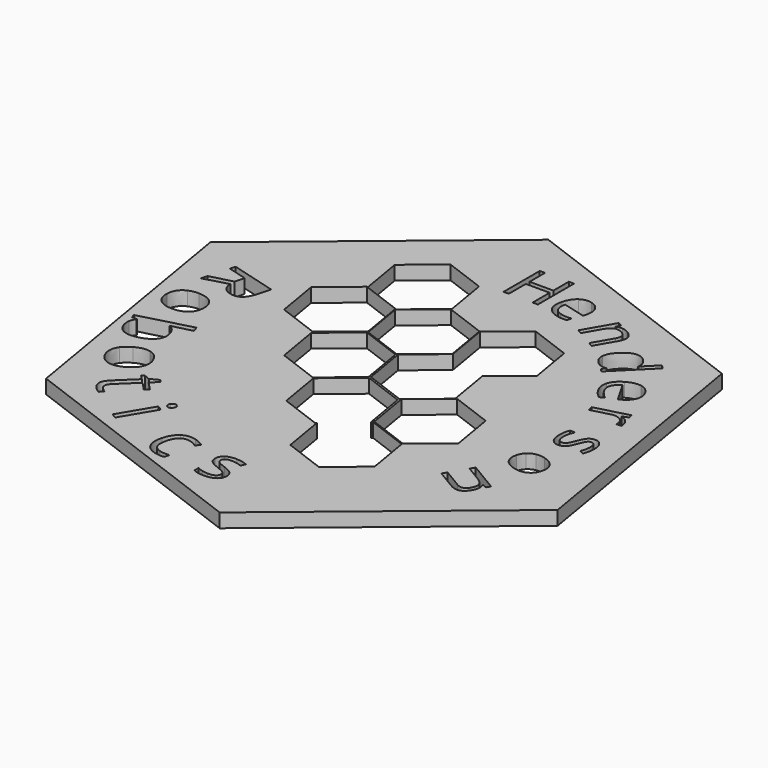
from build123d import *

# Parameters (mm, degrees)
F1_DEPTH = 6.35


with BuildPart() as f1:
    # F0 (on Top) → F1 (new body)
    with BuildSketch(Plane.XY):
        Polygon((112.5371310165, -18.0102200831), (92.5793495724, 100.4138352002), (-19.9577814441, 142.341917108), (-112.5371310165, 65.8459437326), (-92.5793495724, -52.5781115507), (19.9577814441, -94.5061934585), align=None)
        with BuildLine():
            add(Edge.make_bspline(
                [(-72.967737569, -43.6153682612), (-73.0631727177, -44.8083966458), (-72.1048965995, -45.8071760261)],
                knots=[0, 0, 0, 1, 1, 1], degree=2))
            add(Edge.make_bspline(
                [(-72.1048965995, -45.8071760261), (-71.5883258796, -46.3455805358), (-71.0311581814, -46.7701049042)],
                knots=[0, 0, 0, 1, 1, 1], degree=2))
            add(Edge.make_bspline(
                [(-71.0311581814, -46.7701049042), (-70.4739904832, -47.1946292726), (-70.1074129237, -47.4048885653)],
                knots=[0, 0, 0, 1, 1, 1], degree=2))
            Line((-70.1074129237, -47.4048885653), (-71.6563012596, -48.8909652017))
            add(Edge.make_bspline(
                [(-71.6563012596, -48.8909652017), (-72.126794889, -48.712971361), (-72.84603054, -48.1741965048)],
                knots=[0, 0, 0, 1, 1, 1], degree=2))
            add(Edge.make_bspline(
                [(-72.84603054, -48.1741965048), (-73.565266191, -47.6354216486), (-74.0593773144, -47.1204260307)],
                knots=[0, 0, 0, 1, 1, 1], degree=2))
            add(Edge.make_bspline(
                [(-74.0593773144, -47.1204260307), (-77.7764405384, -43.24625445), (-73.6915889323, -39.3270548574)],
                knots=[0, 0, 0, 1, 1, 1], degree=2))
            Line((-73.6915889323, -39.3270548574), (-65.7403687094, -31.6982785728))
            Line((-65.7403687094, -31.6982785728), (-67.5783123579, -29.7826509333))
            Line((-67.5783123579, -29.7826509333), (-66.6029418693, -28.8468344116))
            Line((-66.6029418693, -28.8468344116), (-63.9222781187, -29.9539165765))
            Line((-63.9222781187, -29.9539165765), (-60.2542628032, -28.0681121332))
            Line((-60.2542628032, -28.0681121332), (-59.1312829772, -29.2385567195))
            Line((-59.1312829772, -29.2385567195), (-62.2290596489, -32.2107099923))
            Line((-62.2290596489, -32.2107099923), (-58.5082531589, -36.0887830548))
            Line((-58.5082531589, -36.0887830548), (-60.0805503864, -37.5973192877))
            Line((-60.0805503864, -37.5973192877), (-63.8013568765, -33.7192462252))
            Line((-63.8013568765, -33.7192462252), (-71.6667444964, -41.2656706558))
            add(Edge.make_bspline(
                [(-71.6667444964, -41.2656706558), (-72.8723024203, -42.4223398765), (-72.967737569, -43.6153682612)],
                knots=[0, 0, 0, 1, 1, 1], degree=2))
        make_face(mode=Mode.SUBTRACT)
        with BuildLine():
            add(Edge.make_bspline(
                [(3.4055142751, -68.3015490873), (4.4394744841, -69.3937738183), (4.435601775, -71.0454177006)],
                knots=[0, 0, 0, 1, 1, 1], degree=2))
            add(Edge.make_bspline(
                [(4.435601775, -71.0454177006), (4.4301731682, -73.3606252541), (2.7029292089, -74.6134783422)],
                knots=[0, 0, 0, 1, 1, 1], degree=2))
            add(Edge.make_bspline(
                [(2.7029292089, -74.6134783422), (0.9756852496, -75.8663314303), (-2.143548358, -75.859017575)],
                knots=[0, 0, 0, 1, 1, 1], degree=2))
            add(Edge.make_bspline(
                [(-2.143548358, -75.859017575), (-5.4419925922, -75.8512835138), (-7.2849245981, -74.8007539515)],
                knots=[0, 0, 0, 1, 1, 1], degree=2))
            Line((-7.2849245981, -74.8007539515), (-7.2794619205, -72.4710158066))
            add(Edge.make_bspline(
                [(-7.2794619205, -72.4710158066), (-6.0845295149, -73.0792622713), (-4.7170441834, -73.4287830276)],
                knots=[0, 0, 0, 1, 1, 1], degree=2))
            add(Edge.make_bspline(
                [(-4.7170441834, -73.4287830276), (-3.3495588518, -73.7783037839), (-2.0757103443, -73.7812906533)],
                knots=[0, 0, 0, 1, 1, 1], degree=2))
            add(Edge.make_bspline(
                [(-2.0757103443, -73.7812906533), (-0.109236983, -73.7859015621), (0.9505451405, -73.1611458558)],
                knots=[0, 0, 0, 1, 1, 1], degree=2))
            add(Edge.make_bspline(
                [(0.9505451405, -73.1611458558), (2.010327264, -72.5363901496), (2.0133482042, -71.2480110508)],
                knots=[0, 0, 0, 1, 1, 1], degree=2))
            add(Edge.make_bspline(
                [(2.0133482042, -71.2480110508), (2.0156195878, -70.2793049614), (1.1793015029, -69.5895588912)],
                knots=[0, 0, 0, 1, 1, 1], degree=2))
            add(Edge.make_bspline(
                [(1.1793015029, -69.5895588912), (0.342983418, -68.8998128209), (-2.095952685, -67.9544440275)],
                knots=[0, 0, 0, 1, 1, 1], degree=2))
            add(Edge.make_bspline(
                [(-2.095952685, -67.9544440275), (-4.4091387071, -67.0868670012), (-5.383599622, -66.4403890328)],
                knots=[0, 0, 0, 1, 1, 1], degree=2))
            add(Edge.make_bspline(
                [(-5.383599622, -66.4403890328), (-6.3580605369, -65.7939110644), (-6.8332346452, -64.9766575277)],
                knots=[0, 0, 0, 1, 1, 1], degree=2))
            add(Edge.make_bspline(
                [(-6.8332346452, -64.9766575277), (-7.3084087535, -64.159403991), (-7.3057512346, -63.0260178664)],
                knots=[0, 0, 0, 1, 1, 1], degree=2))
            add(Edge.make_bspline(
                [(-7.3057512346, -63.0260178664), (-7.3009926859, -60.9965786093), (-5.646594751, -59.825895185)],
                knots=[0, 0, 0, 1, 1, 1], degree=2))
            add(Edge.make_bspline(
                [(-5.646594751, -59.825895185), (-3.992196816, -58.6552117608), (-1.1199832611, -58.6619464132)],
                knots=[0, 0, 0, 1, 1, 1], degree=2))
            add(Edge.make_bspline(
                [(-1.1199832611, -58.6619464132), (1.5584890759, -58.6682267889), (4.1181613756, -59.7640289491)],
                knots=[0, 0, 0, 1, 1, 1], degree=2))
            Line((4.1181613756, -59.7640289491), (3.2173156235, -61.8058977678))
            add(Edge.make_bspline(
                [(3.2173156235, -61.8058977678), (0.7253051101, -60.7732205003), (-1.3041341471, -60.7684619516)],
                knots=[0, 0, 0, 1, 1, 1], degree=2))
            add(Edge.make_bspline(
                [(-1.3041341471, -60.7684619516), (-3.0913968819, -60.7642712488), (-4.0008705647, -61.3215695932)],
                knots=[0, 0, 0, 1, 1, 1], degree=2))
            add(Edge.make_bspline(
                [(-4.0008705647, -61.3215695932), (-4.9103442475, -61.8788679377), (-4.9126497018, -62.8621046184)],
                knots=[0, 0, 0, 1, 1, 1], degree=2))
            add(Edge.make_bspline(
                [(-4.9126497018, -62.8621046184), (-4.9142169565, -63.53051182), (-4.5738440026, -63.9987131708)],
                knots=[0, 0, 0, 1, 1, 1], degree=2))
            add(Edge.make_bspline(
                [(-4.5738440026, -63.9987131708), (-4.2334710488, -64.4669145217), (-3.4788740294, -64.892495115)],
                knots=[0, 0, 0, 1, 1, 1], degree=2))
            add(Edge.make_bspline(
                [(-3.4788740294, -64.892495115), (-2.7242770101, -65.3180757083), (-0.5756347401, -66.1271442341)],
                knots=[0, 0, 0, 1, 1, 1], degree=2))
            add(Edge.make_bspline(
                [(-0.5756347401, -66.1271442341), (2.3715540661, -67.2093243564), (3.4055142751, -68.3015490873)],
                knots=[0, 0, 0, 1, 1, 1], degree=2))
        make_face(mode=Mode.SUBTRACT)
        Polygon((-45.7921878886, -45.7525988365), (-54.6549116375, -60.6645132283), (-56.9145564752, -59.3215194689), (-48.0518327263, -44.4096050772), align=None, mode=Mode.SUBTRACT)
        with BuildLine():
            add(Edge.make_bspline(
                [(-46.1364735974, -41.6181544447), (-46.294896449, -41.0173039437), (-45.8420565495, -40.2553813106)],
                knots=[0, 0, 0, 1, 1, 1], degree=2))
            add(Edge.make_bspline(
                [(-45.8420565495, -40.2553813106), (-45.3814536802, -39.4803971466), (-44.7857168684, -39.3454480761)],
                knots=[0, 0, 0, 1, 1, 1], degree=2))
            add(Edge.make_bspline(
                [(-44.7857168684, -39.3454480761), (-44.1899800566, -39.2104990056), (-43.615272699, -39.5520696727)],
                knots=[0, 0, 0, 1, 1, 1], degree=2))
            add(Edge.make_bspline(
                [(-43.615272699, -39.5520696727), (-43.0710422467, -39.8755267438), (-42.8956763794, -40.477609449)],
                knots=[0, 0, 0, 1, 1, 1], degree=2))
            add(Edge.make_bspline(
                [(-42.8956763794, -40.477609449), (-42.720310512, -41.0796921542), (-43.1731504116, -41.8416147874)],
                knots=[0, 0, 0, 1, 1, 1], degree=2))
            add(Edge.make_bspline(
                [(-43.1731504116, -41.8416147874), (-43.6259903112, -42.6035374206), (-44.2425516236, -42.7437850522)],
                knots=[0, 0, 0, 1, 1, 1], degree=2))
            add(Edge.make_bspline(
                [(-44.2425516236, -42.7437850522), (-44.8591129359, -42.8840326839), (-45.4033433882, -42.5605756127)],
                knots=[0, 0, 0, 1, 1, 1], degree=2))
            add(Edge.make_bspline(
                [(-45.4033433882, -42.5605756127), (-45.9780507458, -42.2190049456), (-46.1364735974, -41.6181544447)],
                knots=[0, 0, 0, 1, 1, 1], degree=2))
        make_face(mode=Mode.SUBTRACT)
        with BuildLine():
            add(Edge.make_bspline(
                [(-22.1531029202, -73.3679597217), (-24.046773454, -73.7883237584), (-26.5742108863, -73.109078064)],
                knots=[0, 0, 0, 1, 1, 1], degree=2))
            add(Edge.make_bspline(
                [(-26.5742108863, -73.109078064), (-30.1765355025, -72.1409577638), (-31.5560373116, -69.3924930371)],
                knots=[0, 0, 0, 1, 1, 1], degree=2))
            add(Edge.make_bspline(
                [(-31.5560373116, -69.3924930371), (-32.9355391206, -66.6440283103), (-31.845102546, -62.5865712829)],
                knots=[0, 0, 0, 1, 1, 1], degree=2))
            add(Edge.make_bspline(
                [(-31.845102546, -62.5865712829), (-30.7273399952, -58.4274357382), (-28.1101195997, -56.6959782374)],
                knots=[0, 0, 0, 1, 1, 1], degree=2))
            add(Edge.make_bspline(
                [(-28.1101195997, -56.6959782374), (-25.4928992043, -54.9645207366), (-21.7888960707, -55.9599670129)],
                knots=[0, 0, 0, 1, 1, 1], degree=2))
            add(Edge.make_bspline(
                [(-21.7888960707, -55.9599670129), (-20.5929630328, -56.2813725427), (-19.4666461724, -56.8618162001)],
                knots=[0, 0, 0, 1, 1, 1], degree=2))
            add(Edge.make_bspline(
                [(-19.4666461724, -56.8618162001), (-18.340329312, -57.4422598575), (-17.7561615907, -57.9730450919)],
                knots=[0, 0, 0, 1, 1, 1], degree=2))
            Line((-17.7561615907, -57.9730450919), (-19.0985574859, -59.8965554459))
            add(Edge.make_bspline(
                [(-19.0985574859, -59.8965554459), (-19.8415676113, -59.3386561312), (-20.7659042827, -58.8566224905)],
                knots=[0, 0, 0, 1, 1, 1], degree=2))
            add(Edge.make_bspline(
                [(-20.7659042827, -58.8566224905), (-21.6902409542, -58.3745888499), (-22.4455670834, -58.1715958837)],
                knots=[0, 0, 0, 1, 1, 1], degree=2))
            add(Edge.make_bspline(
                [(-22.4455670834, -58.1715958837), (-27.5004419481, -56.8131044948), (-29.2323883453, -63.2575857638)],
                knots=[0, 0, 0, 1, 1, 1], degree=2))
            add(Edge.make_bspline(
                [(-29.2323883453, -63.2575857638), (-30.0534688687, -66.3127831198), (-29.2603895494, -68.2780669563)],
                knots=[0, 0, 0, 1, 1, 1], degree=2))
            add(Edge.make_bspline(
                [(-29.2603895494, -68.2780669563), (-28.4673102302, -70.2433507928), (-26.0463931494, -70.8939692741)],
                knots=[0, 0, 0, 1, 1, 1], degree=2))
            add(Edge.make_bspline(
                [(-26.0463931494, -70.8939692741), (-23.9740881282, -71.4508986941), (-21.5558351544, -71.1455578415)],
                knots=[0, 0, 0, 1, 1, 1], degree=2))
            Line((-21.5558351544, -71.1455578415), (-22.1531029202, -73.3679597217))
        make_face(mode=Mode.SUBTRACT)
        with BuildLine():
            add(Edge.make_bspline(
                [(-71.4948339907, -23.0783226482), (-72.561892733, -26.0609442778), (-76.1022720551, -28.0076234528)],
                knots=[0, 0, 0, 1, 1, 1], degree=2))
            add(Edge.make_bspline(
                [(-76.1022720551, -28.0076234528), (-79.7425639224, -30.0092395861), (-82.7932065522, -29.3020526751)],
                knots=[0, 0, 0, 1, 1, 1], degree=2))
            add(Edge.make_bspline(
                [(-82.7932065522, -29.3020526751), (-85.843849182, -28.5948657642), (-87.6209403553, -25.3629121254)],
                knots=[0, 0, 0, 1, 1, 1], degree=2))
            add(Edge.make_bspline(
                [(-87.6209403553, -25.3629121254), (-88.7196795215, -23.3646612196), (-88.6316989727, -21.3022590841)],
                knots=[0, 0, 0, 1, 1, 1], degree=2))
            add(Edge.make_bspline(
                [(-88.6316989727, -21.3022590841), (-88.5437184239, -19.2398569486), (-87.2564581701, -17.4345252971)],
                knots=[0, 0, 0, 1, 1, 1], degree=2))
            add(Edge.make_bspline(
                [(-87.2564581701, -17.4345252971), (-85.9691979163, -15.6291936455), (-83.6190810902, -14.3369808435)],
                knots=[0, 0, 0, 1, 1, 1], degree=2))
            add(Edge.make_bspline(
                [(-83.6190810902, -14.3369808435), (-79.9831332465, -12.3377532736), (-76.9514940964, -13.0412458155)],
                knots=[0, 0, 0, 1, 1, 1], degree=2))
            add(Edge.make_bspline(
                [(-76.9514940964, -13.0412458155), (-73.9198549462, -13.7447383575), (-72.142763773, -16.9766919963)],
                knots=[0, 0, 0, 1, 1, 1], degree=2))
            add(Edge.make_bspline(
                [(-72.142763773, -16.9766919963), (-70.4277752483, -20.0957010186), (-71.4948339907, -23.0783226482)],
                knots=[0, 0, 0, 1, 1, 1], degree=2))
        make_face(mode=Mode.SUBTRACT)
        with BuildLine():
            Line((-74.547481639, 8.9194912074), (-75.7870057133, 8.5857765521))
            Line((-75.7870057133, 8.5857765521), (-80.2644527998, 7.3803221831))
            add(Edge.make_bspline(
                [(-80.2644527998, 7.3803221831), (-82.1846199325, 6.8633593213), (-83.7407325732, 6.5740920086)],
                knots=[0, 0, 0, 1, 1, 1], degree=2))
            Line((-83.7407325732, 6.5740920086), (-83.7081782368, 6.4531746829))
            add(Edge.make_bspline(
                [(-83.7081782368, 6.4531746829), (-80.7604046149, 5.3690046154), (-79.8319549412, 1.9204424854)],
                knots=[0, 0, 0, 1, 1, 1], degree=2))
            add(Edge.make_bspline(
                [(-79.8319549412, 1.9204424854), (-78.9529878588, -1.3443253095), (-80.6963415598, -3.751132119)],
                knots=[0, 0, 0, 1, 1, 1], degree=2))
            add(Edge.make_bspline(
                [(-80.6963415598, -3.751132119), (-82.4396952609, -6.1579389284), (-86.5170274847, -7.2556711513)],
                knots=[0, 0, 0, 1, 1, 1], degree=2))
            add(Edge.make_bspline(
                [(-86.5170274847, -7.2556711513), (-90.5991964016, -8.3547055476), (-93.3506186988, -7.1424567124)],
                knots=[0, 0, 0, 1, 1, 1], degree=2))
            add(Edge.make_bspline(
                [(-93.3506186988, -7.1424567124), (-96.102040996, -5.9302078772), (-96.9731950376, -2.6944602404)],
                knots=[0, 0, 0, 1, 1, 1], degree=2))
            add(Edge.make_bspline(
                [(-96.9731950376, -2.6944602404), (-97.4094231452, -1.0741680756), (-97.1721425165, 0.4239959688)],
                knots=[0, 0, 0, 1, 1, 1], degree=2))
            add(Edge.make_bspline(
                [(-97.1721425165, 0.4239959688), (-96.9348618877, 1.9221600132), (-95.9353382153, 3.1612801877)],
                knots=[0, 0, 0, 1, 1, 1], degree=2))
            Line((-95.9353382153, 3.1612801877), (-95.9848208066, 3.3450745229))
            Line((-95.9848208066, 3.3450745229), (-98.2597393392, 3.2980155693))
            Line((-98.2597393392, 3.2980155693), (-98.7441478646, 5.0972653762))
            Line((-98.7441478646, 5.0972653762), (-76.4598394845, 11.0968263711))
            Line((-76.4598394845, 11.0968263711), (-75.2233096623, 11.4297348897))
            Line((-75.2233096623, 11.4297348897), (-74.547481639, 8.9194912074))
        make_face(mode=Mode.SUBTRACT)
        Polygon((-3.2903466672, 19.5115212872), (15.2522997676, 12.6052844447), (18.4983979383, -6.6438464109), (19.0837242934, -6.1601026273), (37.6263707282, -13.0663394699), (40.9167173954, -32.5778607571), (25.6644176278, -45.1831452018), (7.121771193, -38.2769083592), (3.8756730223, -19.0277775036), (3.2903466672, -19.5115212872), (-15.2522997676, -12.6052844447), (-18.5426464348, 6.9062368426), align=None, mode=Mode.SUBTRACT)
        Polygon((49.7063692499, 19.6015298515), (52.9967159171, 0.0900085643), (37.7444161495, -12.5152758804), (19.2017697146, -5.6090390378), (15.9114230474, 13.9024822494), (31.1637228151, 26.5077666941), align=None, mode=Mode.SUBTRACT)
        with BuildLine():
            Line((62.722350632, -21.8460348177), (63.9337989853, -19.8183676586))
            Line((63.9337989853, -19.8183676586), (72.5914298611, -24.9909486816))
            add(Edge.make_bspline(
                [(72.5914298611, -24.9909486816), (74.2245028331, -25.9666431165), (75.4759367053, -25.7043955079)],
                knots=[0, 0, 0, 1, 1, 1], degree=2))
            add(Edge.make_bspline(
                [(75.4759367053, -25.7043955079), (76.7273705775, -25.4421478993), (77.677388843, -23.8520505318)],
                knots=[0, 0, 0, 1, 1, 1], degree=2))
            add(Edge.make_bspline(
                [(77.677388843, -23.8520505318), (78.9308527461, -21.7540596562), (78.3794554024, -20.0992570813)],
                knots=[0, 0, 0, 1, 1, 1], degree=2))
            add(Edge.make_bspline(
                [(78.3794554024, -20.0992570813), (77.8280580587, -18.4444545063), (75.2143599288, -16.8828765711)],
                knots=[0, 0, 0, 1, 1, 1], degree=2))
            Line((75.2143599288, -16.8828765711), (68.1937088982, -12.6883241802))
            Line((68.1937088982, -12.6883241802), (69.4051572515, -10.6606570211))
            Line((69.4051572515, -10.6606570211), (82.7861977522, -18.655282474))
            Line((82.7861977522, -18.655282474), (81.8011665285, -20.3039829387))
            Line((81.8011665285, -20.3039829387), (79.7727704605, -19.5374217896))
            Line((79.7727704605, -19.5374217896), (79.7144155302, -19.6350936181))
            add(Edge.make_bspline(
                [(79.7144155302, -19.6350936181), (80.3293828803, -20.8507452151), (80.2033099846, -22.2995917537)],
                knots=[0, 0, 0, 1, 1, 1], degree=2))
            add(Edge.make_bspline(
                [(80.2033099846, -22.2995917537), (80.0772370888, -23.7484382923), (79.2532654728, -25.1275645103)],
                knots=[0, 0, 0, 1, 1, 1], degree=2))
            add(Edge.make_bspline(
                [(79.2532654728, -25.1275645103), (77.8083973983, -27.5459189833), (75.9127591374, -28.0700589712)],
                knots=[0, 0, 0, 1, 1, 1], degree=2))
            add(Edge.make_bspline(
                [(75.9127591374, -28.0700589712), (74.0171208765, -28.5941989592), (71.4503052243, -27.0606313905)],
                knots=[0, 0, 0, 1, 1, 1], degree=2))
            Line((71.4503052243, -27.0606313905), (62.722350632, -21.8460348177))
        make_face(mode=Mode.SUBTRACT)
        with BuildLine():
            add(Edge.make_bspline(
                [(86.1770568848, -2.2785955218), (83.7359495083, -3.4962546919), (80.3751698675, -2.5957365013)],
                knots=[0, 0, 0, 1, 1, 1], degree=2))
            add(Edge.make_bspline(
                [(80.3751698675, -2.5957365013), (76.9195461387, -1.6698049138), (75.4450941098, 0.5881857946)],
                knots=[0, 0, 0, 1, 1, 1], degree=2))
            add(Edge.make_bspline(
                [(75.4450941098, 0.5881857946), (73.9706420808, 2.8461765029), (74.7927102205, 5.9141765676)],
                knots=[0, 0, 0, 1, 1, 1], degree=2))
            add(Edge.make_bspline(
                [(74.7927102205, 5.9141765676), (75.3009781564, 7.811058328), (76.5850430377, 9.0404149205)],
                knots=[0, 0, 0, 1, 1, 1], degree=2))
            add(Edge.make_bspline(
                [(76.5850430377, 9.0404149205), (77.869107919, 10.2697715131), (79.7452977647, 10.6244738683)],
                knots=[0, 0, 0, 1, 1, 1], degree=2))
            add(Edge.make_bspline(
                [(79.7452977647, 10.6244738683), (81.6214876104, 10.9791762234), (83.8523855069, 10.3814089337)],
                knots=[0, 0, 0, 1, 1, 1], degree=2))
            add(Edge.make_bspline(
                [(83.8523855069, 10.3814089337), (87.3038855796, 9.4565822765), (88.7687289663, 7.212215499)],
                knots=[0, 0, 0, 1, 1, 1], degree=2))
            add(Edge.make_bspline(
                [(88.7687289663, 7.212215499), (90.233572353, 4.9678487216), (89.4115042133, 1.8998486569)],
                knots=[0, 0, 0, 1, 1, 1], degree=2))
            add(Edge.make_bspline(
                [(89.4115042133, 1.8998486569), (88.6181642613, -1.0609363518), (86.1770568848, -2.2785955218)],
                knots=[0, 0, 0, 1, 1, 1], degree=2))
        make_face(mode=Mode.SUBTRACT)
        with BuildLine():
            add(Edge.make_bspline(
                [(-85.1180984879, 19.3300737728), (-87.4584878856, 17.3235839335), (-91.3898794736, 17.3855591027)],
                knots=[0, 0, 0, 1, 1, 1], degree=2))
            add(Edge.make_bspline(
                [(-91.3898794736, 17.3855591027), (-95.432218309, 17.4492832644), (-97.669760896, 19.5182904687)],
                knots=[0, 0, 0, 1, 1, 1], degree=2))
            add(Edge.make_bspline(
                [(-97.669760896, 19.5182904687), (-99.9073034829, 21.587297673), (-99.8507273775, 25.1761999325)],
                knots=[0, 0, 0, 1, 1, 1], degree=2))
            add(Edge.make_bspline(
                [(-99.8507273775, 25.1761999325), (-99.8157475274, 27.395144878), (-98.7467367995, 29.0959899931)],
                knots=[0, 0, 0, 1, 1, 1], degree=2))
            add(Edge.make_bspline(
                [(-98.7467367995, 29.0959899931), (-97.6777260716, 30.7968351082), (-95.7189849761, 31.7020056295)],
                knots=[0, 0, 0, 1, 1, 1], degree=2))
            add(Edge.make_bspline(
                [(-95.7189849761, 31.7020056295), (-93.7602438806, 32.6071761509), (-91.150571673, 32.5660368054)],
                knots=[0, 0, 0, 1, 1, 1], degree=2))
            add(Edge.make_bspline(
                [(-91.150571673, 32.5660368054), (-87.113056631, 32.5023886868), (-84.8897953163, 30.4456690954)],
                knots=[0, 0, 0, 1, 1, 1], degree=2))
            add(Edge.make_bspline(
                [(-84.8897953163, 30.4456690954), (-82.6665340015, 28.388949504), (-82.7231101069, 24.8000472444)],
                knots=[0, 0, 0, 1, 1, 1], degree=2))
            add(Edge.make_bspline(
                [(-82.7231101069, 24.8000472444), (-82.7777090903, 21.3365636122), (-85.1180984879, 19.3300737728)],
                knots=[0, 0, 0, 1, 1, 1], degree=2))
        make_face(mode=Mode.SUBTRACT)
        with BuildLine():
            Line((-86.9551316498, 47.5102251238), (-85.7417407996, 51.8623928649))
            Line((-85.7417407996, 51.8623928649), (-94.4095801162, 54.2789993801))
            Line((-94.4095801162, 54.2789993801), (-93.7342021901, 56.701432368))
            Line((-93.7342021901, 56.701432368), (-72.890329644, 50.8901296482))
            Line((-72.890329644, 50.8901296482), (-74.4840180458, 45.1739177199))
            add(Edge.make_bspline(
                [(-74.4840180458, 45.1739177199), (-75.5536844033, 41.3372583172), (-77.53332218, 39.9151582183)],
                knots=[0, 0, 0, 1, 1, 1], degree=2))
            add(Edge.make_bspline(
                [(-77.53332218, 39.9151582183), (-79.5129599567, 38.4930581195), (-82.4645873451, 39.3159762328)],
                knots=[0, 0, 0, 1, 1, 1], degree=2))
            add(Edge.make_bspline(
                [(-82.4645873451, 39.3159762328), (-86.5977780929, 40.4683159711), (-86.8841882796, 45.0665485028)],
                knots=[0, 0, 0, 1, 1, 1], degree=2))
            Line((-86.8841882796, 45.0665485028), (-97.828442386, 42.0162877574))
            Line((-97.828442386, 42.0162877574), (-97.0296903379, 44.8812367525))
            Line((-97.0296903379, 44.8812367525), (-86.9551316498, 47.5102251238))
        make_face(mode=Mode.SUBTRACT)
        Polygon((-3.8754936377, 19.9034995977), (-19.1277934053, 7.2982151531), (-37.6704398402, 14.2044519956), (-40.9607865074, 33.7159732829), (-25.7084867398, 46.3212577275), (-7.1658403049, 39.415020885), align=None, mode=Mode.SUBTRACT)
        Polygon((-29.1757911749, 66.8978677121), (-25.8854445077, 47.3863464248), (-41.1377442753, 34.7810619802), (-59.6803907101, 41.6872988227), (-62.9707373774, 61.19882011), (-47.7184376097, 73.8041045547), align=None, mode=Mode.SUBTRACT)
        Polygon((4.9981049395, 71.9796337144), (8.2884516067, 52.4681124272), (-6.9638481609, 39.8628279825), (-25.5064945957, 46.7690648251), (-28.7968412629, 66.2805861123), (-13.5445414953, 78.885870557), align=None, mode=Mode.SUBTRACT)
        Polygon((-16.7064143599, 98.8550308269), (-13.4160676927, 79.3435095397), (-28.6683674603, 66.738225095), (-47.2110138952, 73.6444619376), (-50.5013605624, 93.1559832248), (-35.2490607947, 105.7612676695), align=None, mode=Mode.SUBTRACT)
        Polygon((27.3264721896, 45.6410835091), (30.6145172825, 26.1432103934), (15.3622175149, 13.5379259488), (-3.1804289199, 20.4441627913), (-6.4707755871, 39.9556840786), (8.558592322, 52.3767261775), (5.2705472291, 71.8745992932), (20.5228469967, 84.4798837378), (39.0654934316, 77.5736468953), (42.3558400988, 58.062125608), align=None, mode=Mode.SUBTRACT)
        with BuildLine():
            add(Edge.make_bspline(
                [(88.0708640482, 50.9387753988), (89.1739242686, 49.9801827882), (89.5492388219, 48.5794898066)],
                knots=[0, 0, 0, 1, 1, 1], degree=2))
            add(Edge.make_bspline(
                [(89.5492388219, 48.5794898066), (89.8149894993, 47.5876947762), (89.8606590671, 46.7560569418)],
                knots=[0, 0, 0, 1, 1, 1], degree=2))
            Line((89.8606590671, 46.7560569418), (87.6843982847, 46.5086146889))
            add(Edge.make_bspline(
                [(87.6843982847, 46.5086146889), (87.6417457531, 47.4855920059), (87.4517573302, 48.1946384531)],
                knots=[0, 0, 0, 1, 1, 1], degree=2))
            add(Edge.make_bspline(
                [(87.4517573302, 48.1946384531), (86.9668789012, 50.0042293858), (85.1549171792, 50.8940920188)],
                knots=[0, 0, 0, 1, 1, 1], degree=2))
            add(Edge.make_bspline(
                [(85.1549171792, 50.8940920188), (83.3429554572, 51.7839546518), (81.1549164208, 51.197671359)],
                knots=[0, 0, 0, 1, 1, 1], degree=2))
            Line((81.1549164208, 51.197671359), (73.1596564827, 49.0553479153))
            Line((73.1596564827, 49.0553479153), (72.5547240195, 51.312986603))
            Line((72.5547240195, 51.312986603), (87.4533993667, 55.3050746306))
            Line((87.4533993667, 55.3050746306), (87.9522646735, 53.4432839594))
            Line((87.9522646735, 53.4432839594), (85.2643128812, 52.4433118922))
            Line((85.2643128812, 52.4433118922), (85.2934522099, 52.3345624371))
            add(Edge.make_bspline(
                [(85.2934522099, 52.3345624371), (86.9678038278, 51.8973680094), (88.0708640482, 50.9387753988)],
                knots=[0, 0, 0, 1, 1, 1], degree=2))
        make_face(mode=Mode.SUBTRACT)
        with BuildLine():
            add(Edge.make_bspline(
                [(84.1783310039, 22.1919157172), (83.1275106211, 21.1924687754), (81.5349339521, 21.1924687754)],
                knots=[0, 0, 0, 1, 1, 1], degree=2))
            add(Edge.make_bspline(
                [(81.5349339521, 21.1924687754), (79.3025244277, 21.1924687754), (78.0905782529, 22.8551001366)],
                knots=[0, 0, 0, 1, 1, 1], degree=2))
            add(Edge.make_bspline(
                [(78.0905782529, 22.8551001366), (76.8786320781, 24.5177314978), (76.8786320781, 27.525412949)],
                knots=[0, 0, 0, 1, 1, 1], degree=2))
            add(Edge.make_bspline(
                [(76.8786320781, 27.525412949), (76.8786320781, 30.7058959742), (77.8874196456, 32.4852851557)],
                knots=[0, 0, 0, 1, 1, 1], degree=2))
            Line((77.8874196456, 32.4852851557), (80.1338401083, 32.4852851557))
            add(Edge.make_bspline(
                [(80.1338401083, 32.4852851557), (79.5500510068, 31.3317178911), (79.2161236407, 30.0123545216)],
                knots=[0, 0, 0, 1, 1, 1], degree=2))
            add(Edge.make_bspline(
                [(79.2161236407, 30.0123545216), (78.8821962746, 28.6929911521), (78.8821962746, 27.4646988824)],
                knots=[0, 0, 0, 1, 1, 1], degree=2))
            add(Edge.make_bspline(
                [(78.8821962746, 27.4646988824), (78.8821962746, 25.5685518806), (79.4870017838, 24.5480885311)],
                knots=[0, 0, 0, 1, 1, 1], degree=2))
            add(Edge.make_bspline(
                [(79.4870017838, 24.5480885311), (80.091807293, 23.5276251816), (81.3341105011, 23.5276251816)],
                knots=[0, 0, 0, 1, 1, 1], degree=2))
            add(Edge.make_bspline(
                [(81.3341105011, 23.5276251816), (82.2681730636, 23.5276251816), (82.931357483, 24.3355892981)],
                knots=[0, 0, 0, 1, 1, 1], degree=2))
            add(Edge.make_bspline(
                [(82.931357483, 24.3355892981), (83.5945419023, 25.1435534147), (84.5005825879, 27.4973910721)],
                knots=[0, 0, 0, 1, 1, 1], degree=2))
            add(Edge.make_bspline(
                [(84.5005825879, 27.4973910721), (85.3318982685, 29.7298005964), (85.9530498726, 30.6708686281)],
                knots=[0, 0, 0, 1, 1, 1], degree=2))
            add(Edge.make_bspline(
                [(85.9530498726, 30.6708686281), (86.5742014766, 31.6119366598), (87.3611491855, 32.0719624718)],
                knots=[0, 0, 0, 1, 1, 1], degree=2))
            add(Edge.make_bspline(
                [(87.3611491855, 32.0719624718), (88.1480968944, 32.5319882838), (89.2409500925, 32.5319882838)],
                knots=[0, 0, 0, 1, 1, 1], degree=2))
            add(Edge.make_bspline(
                [(89.2409500925, 32.5319882838), (91.1978111609, 32.5319882838), (92.3303620179, 30.9394116148)],
                knots=[0, 0, 0, 1, 1, 1], degree=2))
            add(Edge.make_bspline(
                [(92.3303620179, 30.9394116148), (93.4629128749, 29.3468349458), (93.4629128749, 26.5773394481)],
                knots=[0, 0, 0, 1, 1, 1], degree=2))
            add(Edge.make_bspline(
                [(93.4629128749, 26.5773394481), (93.4629128749, 23.9946564628), (92.4120924921, 21.5240609851)],
                knots=[0, 0, 0, 1, 1, 1], degree=2))
            Line((92.4120924921, 21.5240609851), (90.4412204853, 22.3880688554))
            add(Edge.make_bspline(
                [(90.4412204853, 22.3880688554), (91.4313268015, 24.7932799537), (91.4313268015, 26.7501410221)],
                knots=[0, 0, 0, 1, 1, 1], degree=2))
            add(Edge.make_bspline(
                [(91.4313268015, 26.7501410221), (91.4313268015, 28.4734864499), (90.8919056717, 29.3491701022)],
                knots=[0, 0, 0, 1, 1, 1], degree=2))
            add(Edge.make_bspline(
                [(90.8919056717, 29.3491701022), (90.3524845418, 30.2248537545), (89.4044110409, 30.2248537545)],
                knots=[0, 0, 0, 1, 1, 1], degree=2))
            add(Edge.make_bspline(
                [(89.4044110409, 30.2248537545), (88.7599078728, 30.2248537545), (88.3092226864, 29.8955967013)],
                knots=[0, 0, 0, 1, 1, 1], degree=2))
            add(Edge.make_bspline(
                [(88.3092226864, 29.8955967013), (87.8585375, 29.566339648), (87.4498851289, 28.8377708493)],
                knots=[0, 0, 0, 1, 1, 1], degree=2))
            add(Edge.make_bspline(
                [(87.4498851289, 28.8377708493), (87.0412327578, 28.1092020505), (86.265960831, 26.0355831618)],
                knots=[0, 0, 0, 1, 1, 1], degree=2))
            add(Edge.make_bspline(
                [(86.265960831, 26.0355831618), (85.2291513866, 23.1913626591), (84.1783310039, 22.1919157172)],
                knots=[0, 0, 0, 1, 1, 1], degree=2))
        make_face(mode=Mode.SUBTRACT)
        with BuildLine():
            add(Edge.make_bspline(
                [(67.8350967836, 60.6656310959), (67.0422062463, 61.5467535218), (66.2210770082, 62.9689910817)],
                knots=[0, 0, 0, 1, 1, 1], degree=2))
            add(Edge.make_bspline(
                [(66.2210770082, 62.9689910817), (64.4250046979, 66.0798795773), (65.2826695109, 68.9768716372)],
                knots=[0, 0, 0, 1, 1, 1], degree=2))
            add(Edge.make_bspline(
                [(65.2826695109, 68.9768716372), (66.1403343239, 71.8738636972), (69.5053401933, 73.8166507417)],
                knots=[0, 0, 0, 1, 1, 1], degree=2))
            add(Edge.make_bspline(
                [(69.5053401933, 73.8166507417), (72.9031354012, 75.7783687197), (75.8667133251, 75.2597162099)],
                knots=[0, 0, 0, 1, 1, 1], degree=2))
            add(Edge.make_bspline(
                [(75.8667133251, 75.2597162099), (78.830291249, 74.7410637002), (80.458351525, 71.9211805843)],
                knots=[0, 0, 0, 1, 1, 1], degree=2))
            add(Edge.make_bspline(
                [(80.458351525, 71.9211805843), (81.9799253004, 69.2857374978), (81.1315271957, 66.7465809638)],
                knots=[0, 0, 0, 1, 1, 1], degree=2))
            add(Edge.make_bspline(
                [(81.1315271957, 66.7465809638), (80.2831290909, 64.2074244298), (77.4386539711, 62.5651659537)],
                knots=[0, 0, 0, 1, 1, 1], degree=2))
            Line((77.4386539711, 62.5651659537), (76.0942910903, 61.7889976826))
            Line((76.0942910903, 61.7889976826), (70.5120320915, 71.4577538895))
            add(Edge.make_bspline(
                [(70.5120320915, 71.4577538895), (68.0783975646, 69.9652561042), (67.4814439979, 68.0412516613)],
                knots=[0, 0, 0, 1, 1, 1], degree=2))
            add(Edge.make_bspline(
                [(67.4814439979, 68.0412516613), (66.8844904311, 66.1172472183), (68.1268329382, 63.9654468755)],
                knots=[0, 0, 0, 1, 1, 1], degree=2))
            add(Edge.make_bspline(
                [(68.1268329382, 63.9654468755), (69.4354337125, 61.6988838478), (71.6600638706, 60.0322341983)],
                knots=[0, 0, 0, 1, 1, 1], degree=2))
            Line((71.6600638706, 60.0322341983), (69.7623809017, 58.9366064253))
            add(Edge.make_bspline(
                [(69.7623809017, 58.9366064253), (68.6279873209, 59.78450867), (67.8350967836, 60.6656310959)],
                knots=[0, 0, 0, 1, 1, 1], degree=2))
        make_face(mode=Mode.SUBTRACT)
        Polygon((8.2910283688, 121.6674257377), (8.2910283688, 101.09072361), (5.8996453901, 101.09072361), (5.8996453901, 110.7733477235), (-4.9403900709, 110.7733477235), (-4.9403900709, 101.09072361), (-7.3317730496, 101.09072361), (-7.3317730496, 121.6674257377), (-4.9403900709, 121.6674257377), (-4.9403900709, 112.9125321207), (5.8996453901, 112.9125321207), (5.8996453901, 121.6674257377), align=None, mode=Mode.SUBTRACT)
        with BuildLine():
            add(Edge.make_bspline(
                [(21.409565222, 98.0251251396), (20.2831814255, 98.08449324), (18.7736996795, 98.4889576548)],
                knots=[0, 0, 0, 1, 1, 1], degree=2))
            add(Edge.make_bspline(
                [(18.7736996795, 98.4889576548), (15.4719802406, 99.3736507121), (14.099789453, 101.9000258094)],
                knots=[0, 0, 0, 1, 1, 1], degree=2))
            add(Edge.make_bspline(
                [(14.099789453, 101.9000258094), (12.7275986653, 104.4264009067), (13.6845591396, 107.9978260177)],
                knots=[0, 0, 0, 1, 1, 1], degree=2))
            add(Edge.make_bspline(
                [(13.6845591396, 107.9978260177), (14.650844442, 111.6040518606), (16.9939134755, 113.2491552322)],
                knots=[0, 0, 0, 1, 1, 1], degree=2))
            add(Edge.make_bspline(
                [(16.9939134755, 113.2491552322), (19.336982509, 114.8942586039), (22.3298454523, 114.0923233952)],
                knots=[0, 0, 0, 1, 1, 1], degree=2))
            add(Edge.make_bspline(
                [(22.3298454523, 114.0923233952), (25.1269542786, 113.342840344), (26.2646055036, 111.0634752863)],
                knots=[0, 0, 0, 1, 1, 1], degree=2))
            add(Edge.make_bspline(
                [(26.2646055036, 111.0634752863), (27.4022567286, 108.7841102286), (26.5933278989, 105.7651467364)],
                knots=[0, 0, 0, 1, 1, 1], degree=2))
            Line((26.5933278989, 105.7651467364), (26.2110099506, 104.3383167286))
            Line((26.2110099506, 104.3383167286), (15.9491441322, 107.0879753875))
            add(Edge.make_bspline(
                [(15.9491441322, 107.0879753875), (15.3158866849, 104.4462205647), (16.2088120306, 102.7499575631)],
                knots=[0, 0, 0, 1, 1, 1], degree=2))
            add(Edge.make_bspline(
                [(16.2088120306, 102.7499575631), (17.1017373764, 101.0536945615), (19.3855354072, 100.4417527235)],
                knots=[0, 0, 0, 1, 1, 1], degree=2))
            add(Edge.make_bspline(
                [(19.3855354072, 100.4417527235), (21.7911359996, 99.7971739875), (24.4094398115, 100.1726192305)],
                knots=[0, 0, 0, 1, 1, 1], degree=2))
            Line((24.4094398115, 100.1726192305), (23.8697653905, 98.1585268719))
            add(Edge.make_bspline(
                [(23.8697653905, 98.1585268719), (22.5359490184, 97.9657570391), (21.409565222, 98.0251251396)],
                knots=[0, 0, 0, 1, 1, 1], degree=2))
        make_face(mode=Mode.SUBTRACT)
        with BuildLine():
            Line((43.0989453184, 88.1462191951), (41.0747491326, 89.3148894079))
            Line((41.0747491326, 89.3148894079), (46.0646782106, 97.9577000972))
            add(Edge.make_bspline(
                [(46.0646782106, 97.9577000972), (47.0059193453, 99.5879775647), (46.7279251749, 100.8223286011)],
                knots=[0, 0, 0, 1, 1, 1], degree=2))
            add(Edge.make_bspline(
                [(46.7279251749, 100.8223286011), (46.4499310045, 102.0566796375), (44.8625555755, 102.9731512687)],
                knots=[0, 0, 0, 1, 1, 1], degree=2))
            add(Edge.make_bspline(
                [(44.8625555755, 102.9731512687), (42.7681560538, 104.1823533964), (41.1389696506, 103.6122928207)],
                knots=[0, 0, 0, 1, 1, 1], degree=2))
            add(Edge.make_bspline(
                [(41.1389696506, 103.6122928207), (39.5097832474, 103.042232245), (38.0033470772, 100.4330082599)],
                knots=[0, 0, 0, 1, 1, 1], degree=2))
            Line((38.0033470772, 100.4330082599), (33.956910907, 93.4243752235))
            Line((33.956910907, 93.4243752235), (31.9327147212, 94.5930454362))
            Line((31.9327147212, 94.5930454362), (39.6450374162, 107.9511801884))
            Line((39.6450374162, 107.9511801884), (41.2909156251, 107.0009319614))
            Line((41.2909156251, 107.0009319614), (40.5624496324, 104.9825961059))
            Line((40.5624496324, 104.9825961059), (40.6599542657, 104.9263017797))
            add(Edge.make_bspline(
                [(40.6599542657, 104.9263017797), (41.8536824999, 105.55276498), (43.2891081224, 105.4494560816)],
                knots=[0, 0, 0, 1, 1, 1], degree=2))
            add(Edge.make_bspline(
                [(43.2891081224, 105.4494560816), (44.724533745, 105.3461471833), (46.1012991661, 104.5512712967)],
                knots=[0, 0, 0, 1, 1, 1], degree=2))
            add(Edge.make_bspline(
                [(46.1012991661, 104.5512712967), (48.5155138848, 103.157423779), (49.0621675449, 101.2895393803)],
                knots=[0, 0, 0, 1, 1, 1], degree=2))
            add(Edge.make_bspline(
                [(49.0621675449, 101.2895393803), (49.6088212049, 99.4216549815), (48.1294063113, 96.8592332203)],
                knots=[0, 0, 0, 1, 1, 1], degree=2))
            Line((48.1294063113, 96.8592332203), (43.0989453184, 88.1462191951))
        make_face(mode=Mode.SUBTRACT)
        with BuildLine():
            Line((56.7794885542, 76.2772810544), (58.0214388688, 77.9586907111))
            Line((58.0214388688, 77.9586907111), (57.9322732052, 78.0478563747))
            add(Edge.make_bspline(
                [(57.9322732052, 78.0478563747), (55.1267392894, 77.528784833), (52.8466458913, 79.8088782311)],
                knots=[0, 0, 0, 1, 1, 1], degree=2))
            add(Edge.make_bspline(
                [(52.8466458913, 79.8088782311), (50.7066699646, 81.9488541577), (50.9805359315, 84.6015326502)],
                knots=[0, 0, 0, 1, 1, 1], degree=2))
            add(Edge.make_bspline(
                [(50.9805359315, 84.6015326502), (51.2544018983, 87.2542111427), (53.9516632225, 89.9514724669)],
                knots=[0, 0, 0, 1, 1, 1], degree=2))
            add(Edge.make_bspline(
                [(53.9516632225, 89.9514724669), (56.6489245468, 92.6487337912), (59.3366324071, 92.9480756619)],
                knots=[0, 0, 0, 1, 1, 1], degree=2))
            add(Edge.make_bspline(
                [(59.3366324071, 92.9480756619), (62.0243402674, 93.2474175326), (64.1547627301, 91.1169950699)],
                knots=[0, 0, 0, 1, 1, 1], degree=2))
            add(Edge.make_bspline(
                [(64.1547627301, 91.1169950699), (66.3743508565, 88.8974069435), (65.9444449783, 86.0982420037)],
                knots=[0, 0, 0, 1, 1, 1], degree=2))
            Line((65.9444449783, 86.0982420037), (66.0750089858, 85.9676779963))
            Line((66.0750089858, 85.9676779963), (66.7915187827, 86.8243052645))
            Line((66.7915187827, 86.8243052645), (67.5175820435, 87.633165213))
            Line((67.5175820435, 87.633165213), (71.9567582962, 92.0723414657))
            Line((71.9567582962, 92.0723414657), (73.609507561, 90.4195922009))
            Line((73.609507561, 90.4195922009), (58.1233424844, 74.9334271243))
            Line((58.1233424844, 74.9334271243), (56.7794885542, 76.2772810544))
        make_face(mode=Mode.SUBTRACT)
    extrude(amount=F1_DEPTH)


solid = f1.part
